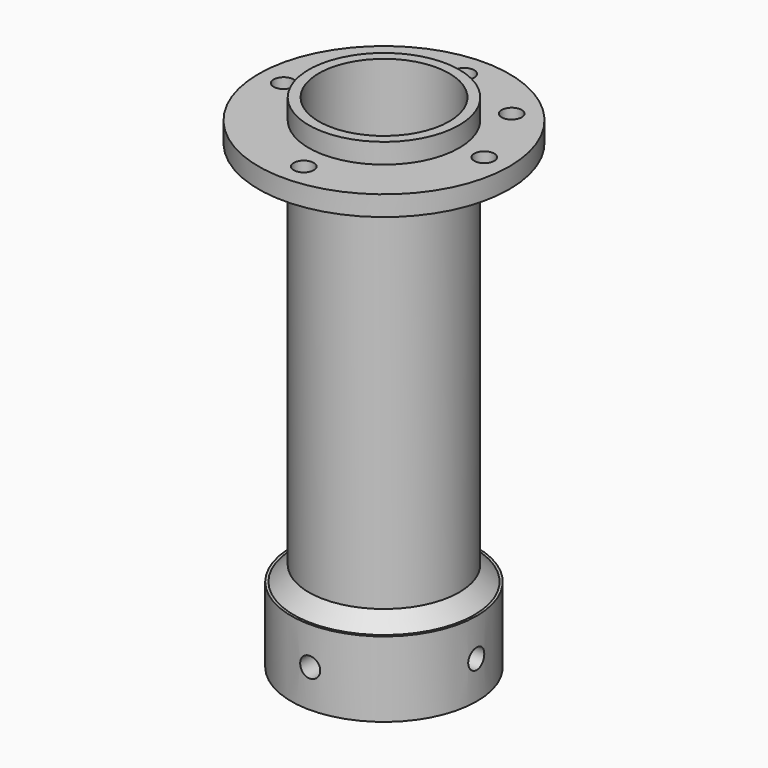
from build123d import *

# Parameters (mm, degrees)
F0_R      = 15
F0_R_2    = 13
F1_DEPTH  = 100
F3_R      = 25
F3_R_2    = 15
F4_DEPTH  = 4
F5_R      = 2
F6_DEPTH  = 96.001
F7_R      = 18.5
F7_R_2    = 13
F8_DEPTH  = 15
F9_R      = 2
F10_DEPTH = 50
F11_R     = 2
F12_DEPTH = 50
F13_SIZE  = 2.99999
F14_SIZE  = 3
F15_R     = 14
F16_DEPTH = 20
F17_R     = 2
F18_DEPTH = 25
F19_R     = 1.5
F20_DEPTH = 6


# Not quite as in the source:
# - a fillet or chamfer is up to 0.001 mm smaller than in the source, because OpenCascade refuses the exact size


with BuildPart() as f1:
    # F0 (on Top) → F1 (new body)
    with BuildSketch(Plane.XY):
        Circle(F0_R)
        Circle(F0_R_2, mode=Mode.SUBTRACT)
    extrude(amount=F1_DEPTH)

    # F3 (on offset) → F4 (join)
    with BuildSketch(Plane.XY.offset(96)):
        Circle(F3_R)
        Circle(F3_R_2, mode=Mode.SUBTRACT)
    extrude(amount=-F4_DEPTH)

    # F5 (on face) → F6 (cut, through all)
    with BuildSketch(Plane.XY.offset(96)):
        with Locations((0, 20)):
            Circle(F5_R)
        with Locations((-20, 0)):
            Circle(F5_R)
        with Locations((0, -20)):
            Circle(F5_R)
        with Locations((20, 0)):
            Circle(F5_R)
    extrude(amount=-F6_DEPTH, mode=Mode.SUBTRACT)

    # F7 (on Top) → F8 (join)
    with BuildSketch(Plane.XY):
        Circle(F7_R)
        Circle(F7_R_2, mode=Mode.SUBTRACT)
    extrude(amount=F8_DEPTH)

    # F9 (on Right) → F10 (cut, symmetric)
    with BuildSketch(Plane.YZ):
        with Locations((0, 7.5)):
            Circle(F9_R)
    extrude(amount=F10_DEPTH, both=True, mode=Mode.SUBTRACT)

    # F11 (on Front) → F12 (cut, symmetric)
    with BuildSketch(Plane.XZ):
        with Locations((0, 7.5)):
            Circle(F11_R)
    extrude(amount=F12_DEPTH, both=True, mode=Mode.SUBTRACT)

    # F13 (size 3 in the source; OpenCascade refuses exactly that, so slightly less here)
    f13_edges = [f1.edges().sort_by_distance(p)[0] for p in [
        (-15, 0, 92),
    ]]
    chamfer(f13_edges, length=F13_SIZE)

    # F14
    f14_edges = [f1.edges().sort_by_distance(p)[0] for p in [
        (-15, 0, 15),
    ]]
    chamfer(f14_edges, length=F14_SIZE)

    # F15 (on face) → F16 (cut)
    with BuildSketch(Plane(origin=(0, 0, 0), x_dir=(1, 0, 0), z_dir=(0, 0, -1))):
        Circle(F15_R)
    extrude(amount=-F16_DEPTH, mode=Mode.SUBTRACT)

    # F17 (on face) → F18 (cut)
    with BuildSketch(Plane.XY.offset(96)):
        with Locations((14.1421356237, 14.1421356237)):
            Circle(F17_R)
    extrude(amount=-F18_DEPTH, mode=Mode.SUBTRACT)

    # F19 (on face) → F20 (cut)
    with BuildSketch(Plane(origin=(0, 0, 0), x_dir=(1, 0, 0), z_dir=(0, 0, -1))):
        with Locations((11.4904851943, -11.4904851943)):
            Circle(F19_R)
    extrude(amount=-F20_DEPTH, mode=Mode.SUBTRACT)


solid = f1.part
